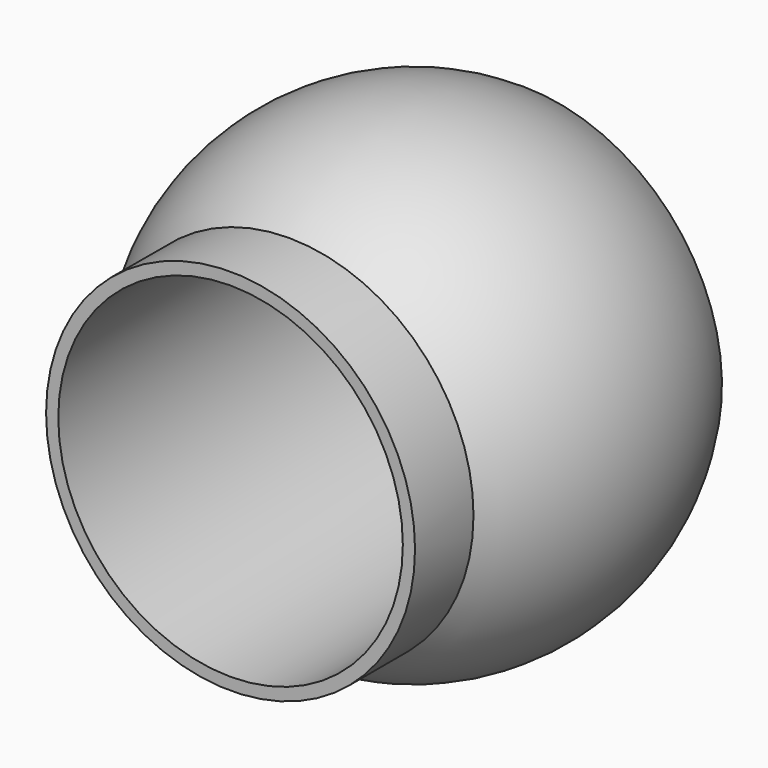
from build123d import *

# Parameters (mm, degrees)
F2_R     = 16.95
F3_DEPTH = 21.02
F4_R     = 15.83
F5_DEPTH = 50
F6_W     = 7.37
F6_H     = 60
F7_DEPTH = 50


with BuildPart() as f1:
    # F0 (on Right) → F1 (revolve)
    with BuildSketch(Plane.YZ):
        with BuildLine():
            Line((-22.18, 0), (22.18, 0))
            ThreePointArc((22.18, 0), (0, 22.18), (-22.18, 0))
        make_face()
    revolve(axis=Axis((0, 3.1962443806, 0), (0, 1, 0)))

    # F2 (on Front) → F3 (join)
    with BuildSketch(Plane.XZ):
        Circle(F2_R)
    extrude(amount=F3_DEPTH)

    # F4 (on face) → F5 (cut, symmetric)
    with BuildSketch(Plane.XZ.offset(21.02)):
        Circle(F4_R)
    extrude(amount=F5_DEPTH, both=True, mode=Mode.SUBTRACT)

    # F6 (on Right) → F7 (cut, symmetric)
    with BuildSketch(Plane.YZ):
        with Locations((16.315, 0)):
            Rectangle(F6_W, F6_H)
    extrude(amount=F7_DEPTH, both=True, mode=Mode.SUBTRACT)


solid = f1.part
